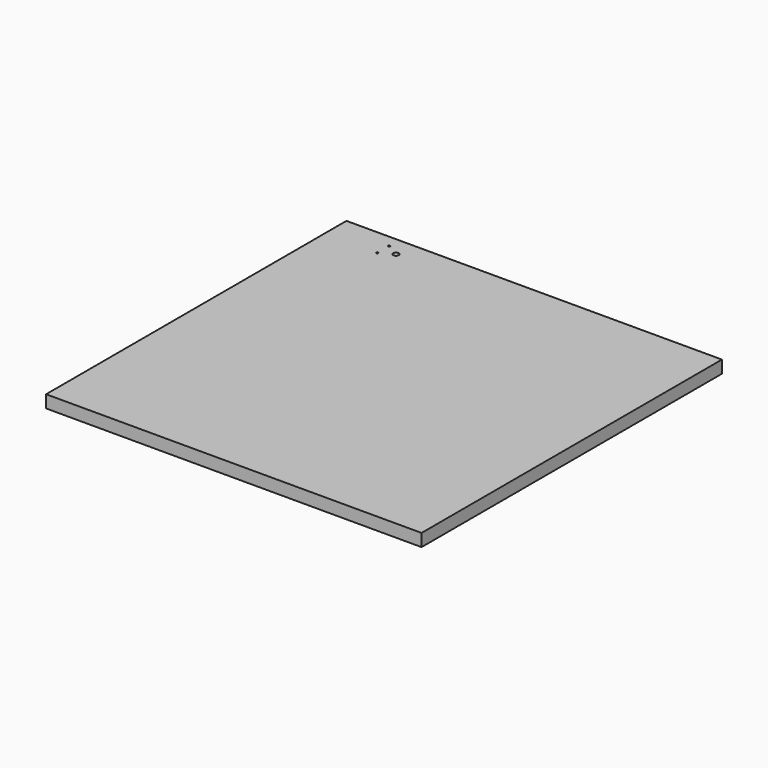
from build123d import *

# Parameters (mm, degrees)
F0_W     = 84
F0_H     = 20
F0_W_2   = 423
F0_W_3   = 9
F0_H_2   = 11.75
F1_DEPTH = 20
F2_D     = 3.3
F3_D     = 8.8


with BuildPart() as f1:
    # F0 (on Top) → F1 (new body)
    with BuildSketch(Plane.XY):
        with Locations((258, -290)):
            Rectangle(F0_W, F0_H)
        with Locations((4.5, -290)):
            Rectangle(F0_W_2, F0_H)
        Polygon((216, -280), (300, -280), (300, 280), (216, 280), (216, 268.25), (216, 256.5), align=None)
        with Locations((-211.5, -290)):
            Rectangle(F0_W_3, F0_H)
        with BuildLine():
            Line((-207, -280), (216, -280))
            Line((216, -280), (216, 256.5))
            Line((216, 256.5), (216, 268.25))
            Line((216, 268.25), (-184.5, 268.25))
            ThreePointArc((-184.5, 268.25), (-195.5, 257.25), (-206.5, 268.25))
            Line((-206.5, 268.25), (-207, 268.25))
            Line((-207, 268.25), (-207, -280))
        make_face()
        with Locations((258, 290)):
            Rectangle(F0_W, F0_H)
        with Locations((-258, -290)):
            Rectangle(F0_W, F0_H)
        Polygon((-216, -280), (-207, -280), (-207, 268.25), (-216, 268.25), (-216, 256.5), align=None)
        Polygon((-207, 280), (216, 280), (216, 300), (-216, 300), (-216, 280), align=None)
        with BuildLine():
            Line((216, 268.25), (216, 280))
            Line((216, 280), (-207, 280))
            Line((-207, 280), (-207, 268.25))
            Line((-207, 268.25), (-206.5, 268.25))
            ThreePointArc((-206.5, 268.25), (-195.5, 279.25), (-184.5, 268.25))
            Line((-184.5, 268.25), (216, 268.25))
        make_face()
        Polygon((-300, -280), (-216, -280), (-216, 256.5), (-216, 268.25), (-216, 280), (-300, 280), align=None)
        with Locations((-211.5, 274.125)):
            Rectangle(F0_W_3, F0_H_2)
        with BuildLine():
            ThreePointArc((-184.5, 268.25), (-195.5, 279.25), (-206.5, 268.25))
            Line((-206.5, 268.25), (-195.5, 268.25))
            Line((-195.5, 268.25), (-184.5, 268.25))
        make_face()
        with BuildLine():
            Line((-195.5, 268.25), (-206.5, 268.25))
            ThreePointArc((-206.5, 268.25), (-195.5, 257.25), (-184.5, 268.25))
            Line((-184.5, 268.25), (-195.5, 268.25))
        make_face()
        with Locations((-258, 290)):
            Rectangle(F0_W, F0_H)
    extrude(amount=F1_DEPTH)

    # F2 (through all)
    with Locations(Plane(origin=(0, 0, 0), x_dir=(1, 0, 0), z_dir=(0, 0, -1))):
        with Locations((-216, -280), (-216, -256.5)):
            Hole(F2_D / 2)

    # F3 (through all)
    with Locations(Plane(origin=(0, 0, 0), x_dir=(1, 0, 0), z_dir=(0, 0, -1))):
        with Locations((-195.5, -268.25)):
            Hole(F3_D / 2)


solid = f1.part
